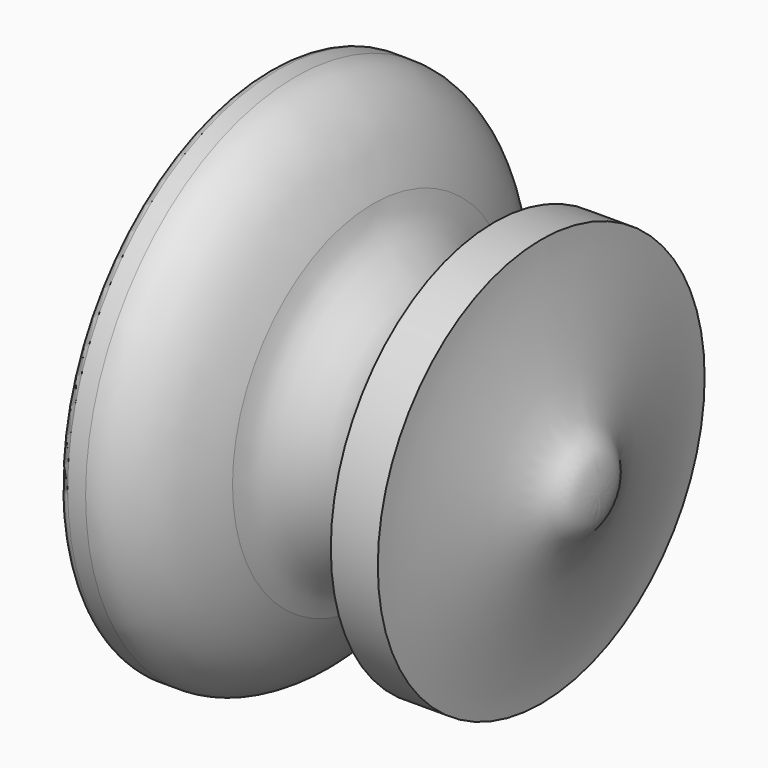
from build123d import *

# Parameters (mm, degrees)
F4_R     = 2.0999999528
F5_DEPTH = 3.5
F6_R     = 0.2
F7_R     = 0.2
F8_R     = 0.2


# Not quite as in the source:
# - ends of sketch curves that miss each other by under 0.0002 mm in the source are joined


with BuildPart() as f2:
    # F1 (on Front) → F2 (revolve)
    with BuildSketch(Plane.XZ):
        with BuildLine():
            Line((45.5202093899, 16.5688355967), (45.5202093899, 14.5688355967))
            add(Edge.make_bspline(
                [(45.5202093899, 14.5688355967), (47.0030293557, 15.1324356496), (50.4613529685, 15.2383481596), (49.5200126524, 9.8090960667), (50.7772336715, 7.0866265215), (51.3850711286, 5.2699102089)],
                knots=[0, 0, 0, 0, 0.3141459464, 0.6391881019, 1, 1, 1, 1], degree=3))
            add(Edge.make_bspline(
                [(51.3850711286, 5.2699102089), (51.9194927912, 3.4284537262), (53.407216137, -1.4620910675), (55.7074866053, -3.3279656709), (55.9983577552, -5.3318521758), (56.1404339969, -6.0311644033)],
                knots=[0, 0, 0, 0, 0.44288519, 0.7345759766, 1, 1, 1, 1], degree=3))
            Line((56.1404339969, -6.0311644033), (57.2202093899, -6.0311644033))
            add(Edge.make_bspline(
                [(50.7202093899, 16.5688355967), (50.8358756015, 14.4597607889), (51.6084715421, 10.0247948502), (52.6677632468, 5.3943286242), (54.7601573389, -1.6439715105), (57.2202093899, -2.029285999), (57.2202093899, -6.0311644033)],
                knots=[0, 0, 0, 0, 0.2620379435, 0.4951606169, 0.7502828141, 1, 1, 1, 1], degree=3))
            Line((50.7202093899, 16.5688355967), (45.5202093899, 16.5688355967))
        make_face()
    revolve(axis=Axis((51.3702093899, 0, -6.0311644033), (-1, 0, 0)))

    # F8
    f8_edges = [f2.edges().sort_by_distance(p)[0] for p in [
        (45.520209, 0, -26.631164),
    ]]
    fillet(f8_edges, radius=F8_R)


with BuildPart() as f3:
    # F0 (on Front) → F3 (revolve)
    with BuildSketch(Plane.XZ):
        with BuildLine():
            Line((36.0297112198, -3.3308526252), (40.5293395695, -3.3308526252))
            Line((40.5293395695, -3.3308526252), (40.5293395695, -2.8304809825))
            ThreePointArc((40.5293395695, -2.8304809825), (40.3830018139, -2.4771903884), (40.0297112198, -2.3308526328))
            Line((40.0297112198, -2.3308526328), (38.2793395695, -2.3308526328))
            Line((38.2793395695, -2.3308526328), (38.2793395695, -1.3308526328))
            Line((38.2793395695, -1.3308526328), (37.8297112198, -1.3308526328))
            ThreePointArc((37.8297112198, -1.3308526328), (37.4758950327, -1.1842971695), (37.3293395695, -0.8304809825))
            Line((37.3293395695, -0.8304809825), (37.3293395695, 0.7649264106))
            ThreePointArc((37.3293395695, 0.7649264106), (37.4738090239, 1.1159109608), (37.823495324, 1.2634950702))
            Line((37.823495324, 1.2634950702), (38.4592522457, 1.2691473748))
            Line((38.4592522457, 1.2691473748), (38.4592522457, 1.569147422))
            Line((38.4592522457, 1.569147422), (37.2592551654, 1.571794543))
            Line((37.2592551654, 1.571794543), (37.2592551654, 4.321794543))
            Line((37.2592551654, 4.321794543), (38.4592522457, 4.319147422))
            add(Edge.make_bspline(
                [(32.1150946415, 14.0060802641), (32.527128629, 11.6368848354), (35.086797429, 9.2444942472), (38.4592522457, 6.1470539947), (38.4592522457, 4.319147422)],
                knots=[0, 0, 0, 0, 0.5052582866, 1, 1, 1, 1], degree=3))
            add(Edge.make_bspline(
                [(23.510220087, 23.5689664246), (25.009952657, 23.5689664246), (28.5696091969, 21.3746279059), (30.5924900929, 17.8711530672), (32.1150946415, 14.0060802641)],
                knots=[0, 0, 0, 0, 0.4257092133, 1, 1, 1, 1], degree=3))
            Line((23.510220087, 23.5689664246), (21.5242667176, 23.5689664246))
            ThreePointArc((21.5242667176, 23.5689664246), (20.8175904861, 23.275592193), (20.5264681652, 22.5679852892))
            Line((20.5264681652, 22.5679852892), (20.5423877116, 17.5689664246))
            Line((20.5423877116, 17.5689664246), (22.0423801057, 17.5737432016))
            Line((22.0423801057, 17.5737432016), (22.0423801057, 19.9737432016))
            ThreePointArc((22.0423801057, 19.9737432016), (22.3352733245, 20.6808499828), (23.0423801057, 20.9737432016))
            Line((23.0423801057, 20.9737432016), (24.6423801057, 20.9737432016))
            ThreePointArc((24.6423801057, 20.9737432016), (25.3494868869, 20.6808499828), (25.6423801057, 19.9737432016))
            Line((25.6423801057, 19.9737432016), (25.6423801057, 17.5689664246))
            Line((25.6423801057, 17.5689664246), (25.9363012909, 17.5689664246))
            ThreePointArc((25.9363012909, 17.5689664246), (26.196917794, 17.4951500251), (26.3801148345, 17.2956289311))
            Line((26.3801148345, 17.2956289311), (32.2518409864, 5.6430637266))
            ThreePointArc((32.2518409864, 5.6430637266), (32.6204651827, 5.2415927055), (33.144870756, 5.093061316))
            Line((33.144870756, 5.093061316), (33.5281772316, 5.093061316))
            ThreePointArc((33.5281772316, 5.093061316), (34.2352840127, 4.8001680972), (34.5281772316, 4.093061316))
            Line((34.5281772316, 4.093061316), (34.5281772316, 1.8878950192))
            ThreePointArc((34.5281772316, 1.8878950192), (34.2355702979, 1.1810746391), (33.5289871321, 0.8878953472))
            Line((33.5289871321, 0.8878953472), (33.5281772316, 0.8878950192))
            ThreePointArc((33.5281772316, 0.8878950192), (32.8215940661, 0.5947153993), (32.5289871324, -0.1121049808))
            Line((32.5289871324, -0.1121049808), (32.5289871324, -0.585266359))
            Line((32.5289871324, -0.585266359), (32.5289871324, -0.785266359))
            Line((32.5289871324, -0.785266359), (32.5289871324, -3.3308526252))
            Line((32.5289871324, -3.3308526252), (36.0297112198, -3.3308526252))
        make_face()
    revolve(axis=Axis((30.5297849349, 0, -5.430852578), (-1, 0, 0)))

    # F4 (on face) → F5 (cut)
    with BuildSketch(Plane(origin=(32.5289871324, 0, 0), x_dir=(0, -1, 0), z_dir=(-1, 0, 0))):
        Polygon((-2.1939310229, -9.2148658602), (2.1939310229, -9.2148658602), (4.3878620458, -5.4148658602), (2.1939310229, -1.6148658602), (-2.1939310229, -1.6148658602), (-4.3878620458, -5.4148658602), align=None)
        with Locations((0, -5.430852578)):
            Circle(F4_R, mode=Mode.SUBTRACT)
    extrude(amount=-F5_DEPTH, mode=Mode.SUBTRACT)

    # F6
    f6_edges = [f3.edges().sort_by_distance(p)[0] for p in [
        (36.028987, 0, -9.214866),
        (36.028987, -3.290897, -7.314866),
        (36.028987, -3.290897, -3.514866),
        (36.028987, 0, -1.614866),
        (36.028987, 3.290897, -3.514866),
        (36.028987, 3.290897, -7.314866),
        (36.028987, 0, -7.530853),
    ]]
    fillet(f6_edges, radius=F6_R)

    # F7
    f7_edges = [f3.edges().sort_by_distance(p)[0] for p in [
        (32.528987, 0, -10.7496),
        (32.528987, 0, -9.214866),
        (32.528987, -3.290897, -7.314866),
        (32.528987, -3.290897, -3.514866),
        (32.528987, 0, -1.614866),
        (32.528987, 3.290897, -3.514866),
        (32.528987, 3.290897, -7.314866),
    ]]
    fillet(f7_edges, radius=F7_R)


solid = Compound([f2.part, f3.part])
